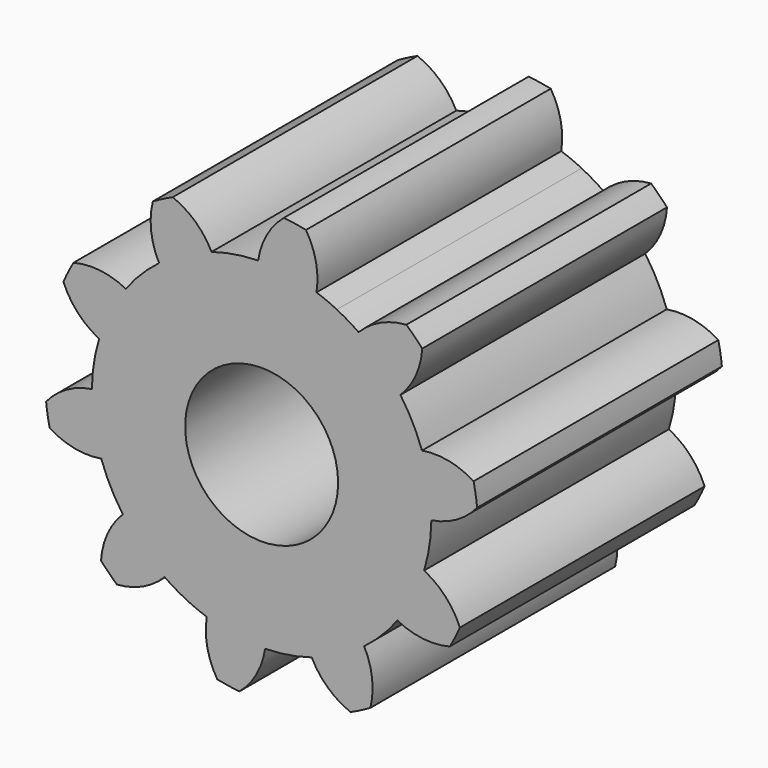
from build123d import *

# Parameters (mm, degrees)
F2_R     = 1.27
F3_DEPTH = 5.08
F4_DEPTH = 5.08
F6_COUNT = 10
F6_ANGLE = 324


# Not quite as in the source:
# - a variable given as a bare number and used for a length is read in inches; the dataset says mm whatever the document's units were


with BuildPart() as f3:
    # F2 (on Front) → F3 (new body)
    with BuildSketch(Plane.XZ):
        with BuildLine():
            ThreePointArc((2.818765, -0.042015), (2.819, -0.021008), (2.819078, 0))
            ThreePointArc((2.819078, 0), (2.779747, 0.469261), (2.662852, 0.925429))
            ThreePointArc((2.662852, 0.925429), (-2.783167, -0.448533), (2.818765, -0.042015))
        make_face()
        Circle(F2_R, mode=Mode.SUBTRACT)
    extrude(amount=F3_DEPTH)

    # F2 (on Front) → F4 (join)
    with BuildSketch(Plane.XZ):
        with BuildLine():
            ThreePointArc((2.662852, 0.925429), (2.779747, 0.469261), (2.819078, 0))
            ThreePointArc((2.819078, 0), (2.819, -0.021008), (2.818765, -0.042015))
            ThreePointArc((2.818765, -0.042015), (3.238382, 0.103424), (3.578985, 0.388415))
            ThreePointArc((3.578985, 0.388415), (3.554141, 0.572783), (3.519806, 0.755621))
            ThreePointArc((3.519806, 0.755621), (3.106915, 0.91918), (2.662852, 0.925429))
        make_face()
    extrude(amount=F4_DEPTH)

    # F6: F3 ×10 about axis
    f6_axis = Axis((0, 6.146542, 0), (0, 1, 0))


with BuildPart() as f3_1:
    add(f3.part)
    for i in range(1, F6_COUNT):
        add(f3.part.rotate(f6_axis, i * F6_ANGLE / (F6_COUNT - 1)))


solid = f3_1.part
